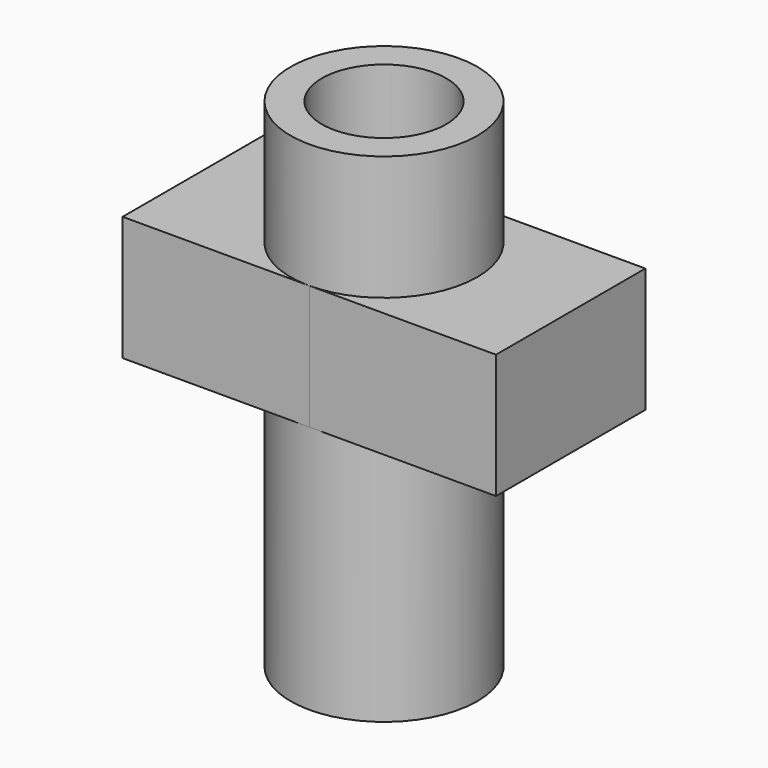
from build123d import *

# Parameters (mm, degrees)
F1_DEPTH = 25.4
F0_R     = 9.525
F2_DEPTH = 50.8
F3_R     = 12.7
F4_DEPTH = 50.801
F5_DEPTH = 50.8


with BuildPart() as f1:
    # F0 (on Top) → F1 (new body)
    with BuildSketch(Plane.XY):
        with BuildLine():
            Line((0, 38.1), (0, 0))
            Line((0, 0), (38.1, 0))
            ThreePointArc((38.1, 0), (19.05, 19.05), (38.1, 38.1))
            Line((38.1, 38.1), (0, 38.1))
        make_face()
    extrude(amount=F1_DEPTH)


with BuildPart() as f1b:
    # F0 (on Top) → F1, piece 2 (new body)
    with BuildSketch(Plane.XY):
        with BuildLine():
            ThreePointArc((57.15, 19.05), (51.5703841816, 5.5796158184), (38.1, 0))
            Line((38.1, 0), (76.2, 0))
            Line((76.2, 0), (76.2, 38.1))
            Line((76.2, 38.1), (38.1, 38.1))
            ThreePointArc((38.1, 38.1), (51.5703841816, 32.5203841816), (57.15, 19.05))
        make_face()
    extrude(amount=F1_DEPTH)


with BuildPart() as f2:
    # F0 (on Top) → F2 (new body)
    with BuildSketch(Plane.XY):
        with BuildLine():
            ThreePointArc((38.1, 38.1), (19.05, 19.05), (38.1, 0))
            ThreePointArc((38.1, 0), (51.5703841816, 5.5796158184), (57.15, 19.05))
            ThreePointArc((57.15, 19.05), (51.5703841816, 32.5203841816), (38.1, 38.1))
        make_face()
        with Locations((38.1, 19.05)):
            Circle(F0_R, mode=Mode.SUBTRACT)
        with Locations((38.1, 19.05)):
            Circle(F0_R)
    extrude(amount=F2_DEPTH)

    # F3 (on face) → F4 (cut, through all)
    with BuildSketch(Plane.XY.offset(50.8)):
        with Locations((38.1, 19.05)):
            Circle(F3_R)
    extrude(amount=-F4_DEPTH, mode=Mode.SUBTRACT)

    # F5 (add): a face of the model
    f5_faces = [f2.faces().sort_by_distance(p)[0] for p in [
        (38.1, 37.5611846327, 0),
    ]]
    extrude(f5_faces, amount=F5_DEPTH)


solid = Compound([f1.part, f1b.part, f2.part])
